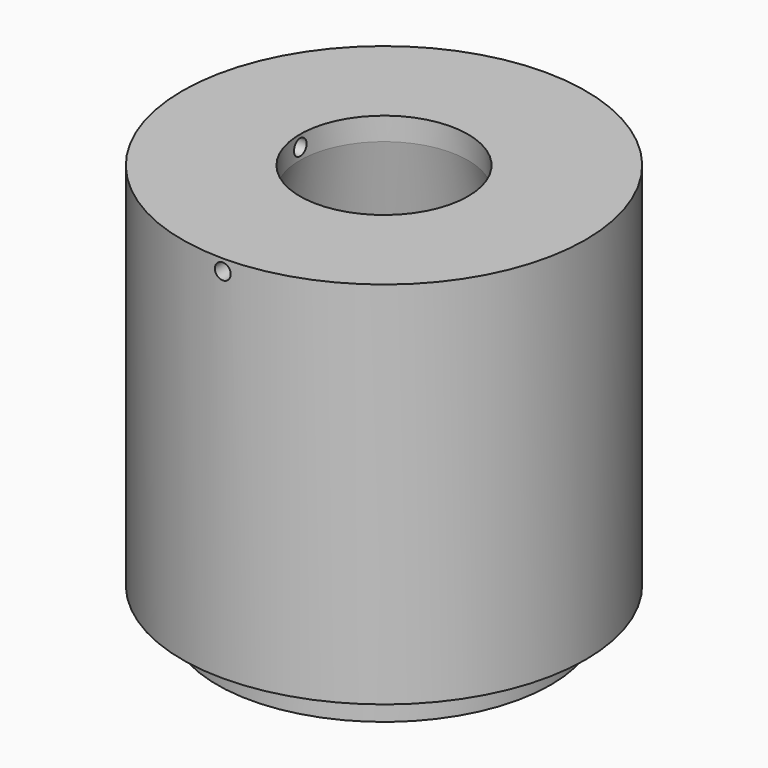
from build123d import *

# Parameters (mm, degrees)
F0_R            = 38.1
F1_DEPTH        = 76.2
F3_R            = 28.575
F4_DEPTH        = 6.35
F5_R            = 1.5
F6_DEPTH        = 50.8
F6_COPIES_COUNT = 2
F6_COPIES_ANGLE = 90
F2_R            = 15.875
F7_DEPTH        = 4.318
F7_FACE_R       = 15.875
F4_FACE_R       = 28.575
F9_R            = 38.1
F9_R_2          = 31.496
F10_DEPTH       = 6.35


# Not quite as in the source:
# - a pattern or mirror of a feature is missing from the dataset's text; its kind, count and spacing are read off the source's solid


with BuildPart() as f1:
    # F0 (on Top) → F1 (new body)
    with BuildSketch(Plane.XY):
        Circle(F0_R)
    extrude(amount=F1_DEPTH)

    # F3 (on face) → F4 (cut)
    with BuildSketch(Plane(origin=(0, 0, 0), x_dir=(1, 0, 0), z_dir=(0, 0, -1))):
        Circle(F3_R)
    extrude(amount=-F4_DEPTH, mode=Mode.SUBTRACT)

    # F5 (on Right) → F6 (cut)
    with BuildSketch(Plane.YZ):
        with Locations((0, 74.041)):
            Circle(F5_R)
    f6 = extrude(amount=-F6_DEPTH, mode=Mode.SUBTRACT)

    # F6_copies: F6 ×2 about axis
    f6_copies_axis = Axis((0, 0, 0), (0, 0, 1))
    for i in range(1, F6_COPIES_COUNT):
        add(f6.rotate(f6_copies_axis, i * F6_COPIES_ANGLE / (F6_COPIES_COUNT - 1)), mode=Mode.SUBTRACT)

    # F2 (on face) → F7 (cut)
    with BuildSketch(Plane.XY.offset(76.2)):
        Circle(F2_R)
    extrude(amount=-F7_DEPTH, mode=Mode.SUBTRACT)

    # F7_face (on face) → F8 section 0
    with BuildSketch(Plane.XY.offset(71.882)):
        Circle(F7_FACE_R)
    # F4_face (on face) → F8 section 1
    with BuildSketch(Plane(origin=(0, 0, 6.35), x_dir=(1, 0, 0), z_dir=(0, 0, -1))):
        Circle(F4_FACE_R)
    loft(mode=Mode.SUBTRACT)

    # F9 (on face) → F10 (cut)
    with BuildSketch(Plane(origin=(0, 0, 0), x_dir=(1, 0, 0), z_dir=(0, 0, -1))):
        Circle(F9_R)
        Circle(F9_R_2, mode=Mode.SUBTRACT)
    extrude(amount=-F10_DEPTH, mode=Mode.SUBTRACT)


solid = f1.part
